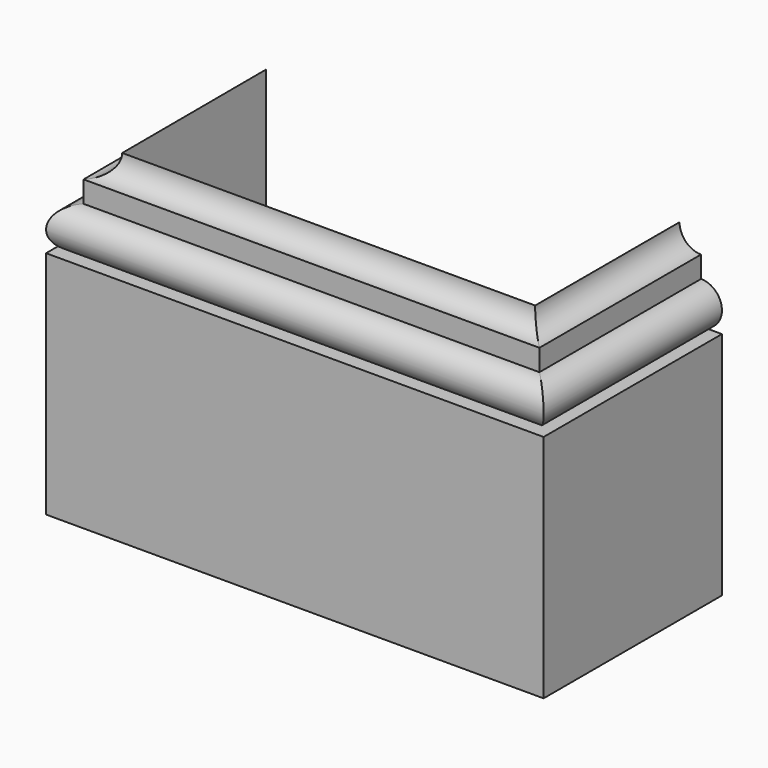
from build123d import *


# Not quite as in the source:
# - the program builds the solid bodies; features that only make, move or delete a surface that nothing else refers to are left out


with BuildPart() as f2:
    # F2: sweep along a path in F1
    with BuildLine(Plane.XY) as f2_path:
        Line((131.5030422138, 92.3344379031), (131.5030422138, -98.4952900969))
        Line((131.5030422138, -98.4952900969), (-316.1564137862, -98.4952900969))
        Line((-316.1564137862, -98.4952900969), (-316.6663944721, 91.8979942799))
    # F0 (on Front) → F2 (sweep)
    with BuildSketch(Plane.XZ):
        with BuildLine():
            Line((223.829728, 92.340303), (197.316539, 92.340303))
            ThreePointArc((197.316539, 92.340303), (223.829728, 118.853492), (197.316539, 145.366681))
            Line((197.316539, 145.366681), (197.316539, 172.683461))
            ThreePointArc((197.316539, 172.683461), (178.0008290346, 180.6842900346), (170, 200))
            Line((170, 200), (170, -200))
            Line((170, -200), (223.829728, -200))
            Line((223.829728, -200), (223.829728, 92.340303))
        make_face()
    sweep(path=f2_path.line, transition=Transition.RIGHT)


solid = f2.part
